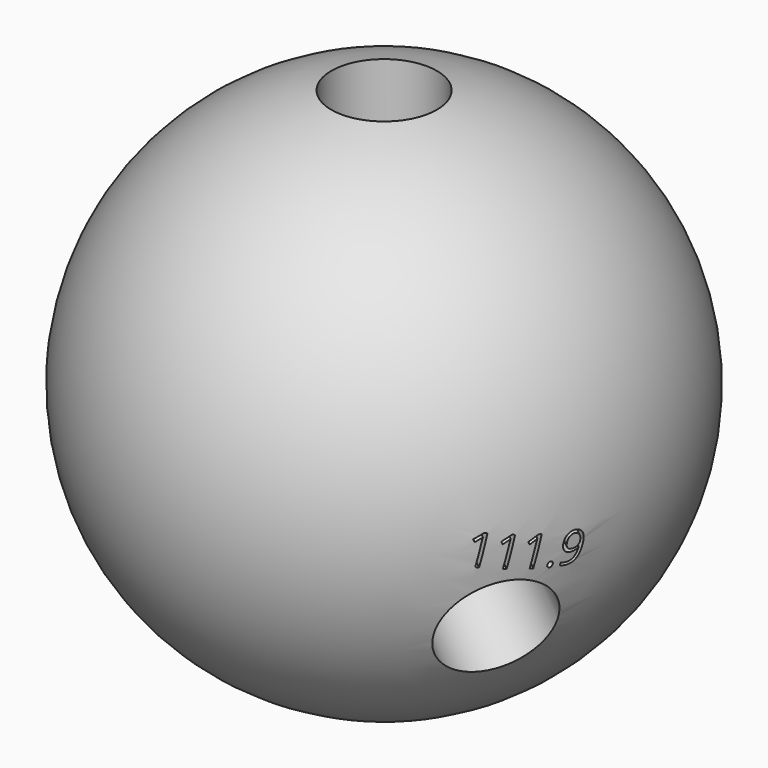
from build123d import *

# Parameters (mm, degrees)
F3_R          = 3.175
F4_DEPTH      = 25.4
F5_DEPTH      = 25.4
F9_ANGLE      = 111.2
F10_ANGLE     = 105.4
F11_ANGLE     = 30
F12_ANGLE     = 111.9
F13_ANGLE     = 60
F15_TEXT_SIZE = 2.4763877887
F16_DEPTH     = 12.7
F18_TEXT_SIZE = 1.9287674351
F19_DEPTH     = 6.35
F21_TEXT_SIZE = 2.2549447345
F22_DEPTH     = 6.35


# Not quite as in the source:
# - Text() gives the source's letters only with a copy of the font that has no kerning and outlines rounded to 1/6400 em; it was checked with that copy


with BuildPart() as f1:
    # F0 (on Front) → F1 (revolve)
    with BuildSketch(Plane.XZ):
        with BuildLine():
            Line((0, -15.875), (0, 15.875))
            ThreePointArc((0, 15.875), (-15.875, 0), (0, -15.875))
        make_face()
    revolve(axis=Axis((0, 0, 0), (0, 0, -1)))

    # F15 (on offset) → F16 (cut)
    with BuildSketch(Plane(origin=(14.9883411744, -8.6535228118, -6.9573877319), x_dir=(0.4207938235, 0.8858780794, -0.1953268712), z_dir=(0.8035297664, -0.4639181269, -0.3729877826))):
        with Locations((-3.0540010697, 3.768344292)):
            Text('111.9', F15_TEXT_SIZE, font='Open Sans', text_align=(TextAlign.LEFT, TextAlign.BOTTOM))
    extrude(amount=-F16_DEPTH, mode=Mode.SUBTRACT)

    # F18 (on offset) → F19 (cut)
    with BuildSketch(Plane(origin=(0, 17.3907524045, -6.7454283088), x_dir=(-1, 0, 0), z_dir=(0, 0.9323238012, -0.3616245701))):
        with Locations((-2.3466406128, 3.6702703219)):
            Text('111.2', F18_TEXT_SIZE, font='Open Sans', text_align=(TextAlign.LEFT, TextAlign.BOTTOM))
    extrude(amount=-F19_DEPTH, mode=Mode.SUBTRACT)

    # F21 (on offset) → F22 (cut)
    with BuildSketch(Plane(origin=(-15.5740743936, -8.9916960436, -4.953451454), x_dir=(0.4593721775, -0.8761449725, 0.1461067748), z_dir=(-0.8349311117, -0.4820477021, -0.2655561175))):
        with Locations((-3.1698929088, 3.948464524)):
            Text('105.4', F21_TEXT_SIZE, font='Open Sans', text_align=(TextAlign.LEFT, TextAlign.BOTTOM))
    extrude(amount=-F22_DEPTH, mode=Mode.SUBTRACT)


with BuildPart() as f4:
    # F3 (on offset) → F4 (new body)
    with BuildSketch(Plane.XY.offset(5.953125)):
        Circle(F3_R)
    extrude(amount=F4_DEPTH)


with BuildPart() as f5:
    # F3 (on offset) → F5 (new body)
    with BuildSketch(Plane.XY.offset(5.953125)):
        Circle(F3_R)
    extrude(amount=F5_DEPTH)


with BuildPart() as f9_1:
    # F9: copy of F5
    add(f5.part.rotate(Axis((-17.6395475864, 0, 0), (-1, 0, 0)), F9_ANGLE))


with BuildPart() as f10_1:
    # F10: copy of F5
    add(f5.part.rotate(Axis((0, -17.3120051622, 0), (0, -1, 0)), F10_ANGLE))


with BuildPart() as f10_1_1:
    # F11: moved
    add(f10_1.part.rotate(Axis((0, 0, 17.7610963583), (0, 0, 1)), F11_ANGLE))


with BuildPart() as f12_1:
    # F12: copy of F5
    add(f5.part.rotate(Axis((14.7991264239, 0, 0), (1, 0, 0)), F12_ANGLE))


with BuildPart() as f12_1_1:
    # F13: moved
    add(f12_1.part.rotate(Axis((0, 0, 17.7610963583), (0, 0, 1)), F13_ANGLE))


with BuildPart() as f1_1:
    add(f1.part)

    # F23: cut F12_1, F10_1, F9_1
    add(f12_1_1.part, mode=Mode.SUBTRACT)
    add(f10_1_1.part, mode=Mode.SUBTRACT)
    add(f9_1.part, mode=Mode.SUBTRACT)

    # F24: cut F5
    add(f5.part, mode=Mode.SUBTRACT)


solid = f1_1.part
